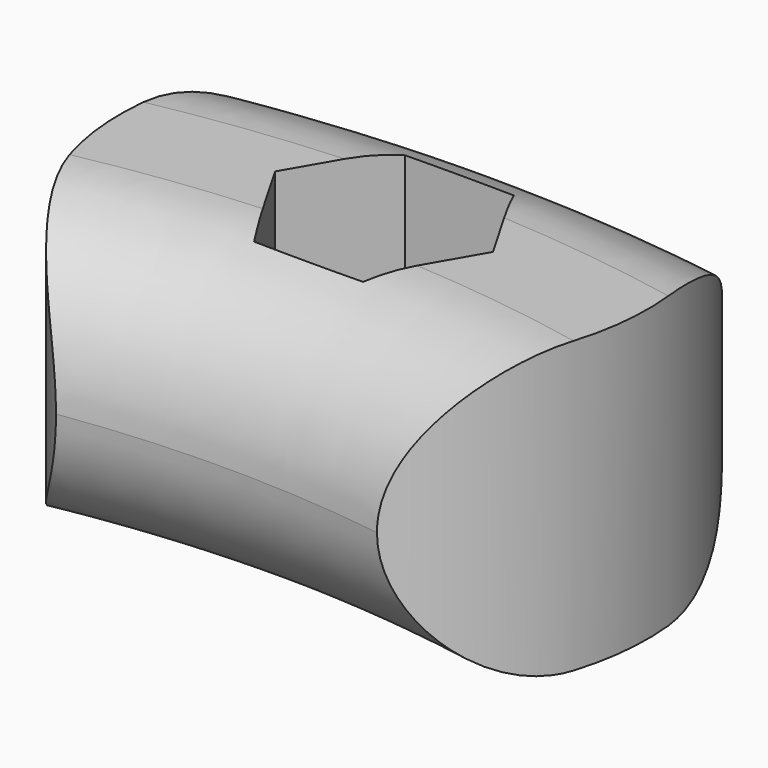
from build123d import *

# Parameters (mm, degrees)
F0_W     = 15
F0_H     = 11
F3_DEPTH = 8.5
F5_R     = 10
F6_DEPTH = 25


# Not quite as in the source:
# - a fillet or chamfer that OpenCascade refuses, or shapes differently, is made with other operations: its cross-section is extruded or revolved along the edge and cut away or added


with BuildPart() as f1:
    # F0 (on Front) → F1 (revolve)
    with BuildSketch(Plane.XZ):
        with Locations((50, 5.5)):
            Rectangle(F0_W, F0_H)
    revolve(axis=Axis((0, 0, 11.3872010261), (0, 0, 1)))

    # F2 (on face) → F3 (cut)
    with BuildSketch(Plane.XY.offset(11)):
        Polygon((-2.0640272124, 46.425), (2.0640272124, 46.425), (4.1280544247, 50), (2.0640272124, 53.575), (-2.0640272124, 53.575), (-4.1280544247, 50), align=None)
        Polygon((-15.8591658515, 43.680976315), (-15.3203466262, 47.7737146618), (-18.5953523929, 50.2867149724), (-22.409177385, 48.7069769362), (-22.9479966103, 44.6142385893), (-19.6729908436, 42.1012382787), align=None)
        Polygon((-31.3679446782, 34.286919955), (-32.4363637825, 38.2743143361), (-36.4237581637, 39.3427334405), (-39.3427334405, 36.4237581637), (-38.2743143361, 32.4363637825), (-34.286919955, 31.3679446782), align=None)
        Polygon((-42.1012382787, 19.6729908436), (-44.6142385893, 22.9479966103), (-48.7069769362, 22.409177385), (-50.2867149724, 18.5953523929), (-47.7737146618, 15.3203466262), (-43.680976315, 15.8591658515), align=None)
        Polygon((-46.425, 2.0640272124), (-50, 4.1280544247), (-53.575, 2.0640272124), (-53.575, -2.0640272124), (-50, -4.1280544247), (-46.425, -2.0640272124), align=None)
        Polygon((-43.680976315, -15.8591658515), (-47.7737146618, -15.3203466262), (-50.2867149724, -18.5953523929), (-48.7069769362, -22.409177385), (-44.6142385893, -22.9479966103), (-42.1012382787, -19.6729908436), align=None)
        Polygon((-34.286919955, -31.3679446782), (-38.2743143361, -32.4363637825), (-39.3427334405, -36.4237581637), (-36.4237581637, -39.3427334405), (-32.4363637825, -38.2743143361), (-31.3679446782, -34.286919955), align=None)
        Polygon((-19.6729908436, -42.1012382787), (-22.9479966103, -44.6142385893), (-22.409177385, -48.7069769362), (-18.5953523929, -50.2867149724), (-15.3203466262, -47.7737146618), (-15.8591658515, -43.680976315), align=None)
        Polygon((-2.0640272124, -46.425), (-4.1280544247, -50), (-2.0640272124, -53.575), (2.0640272124, -53.575), (4.1280544247, -50), (2.0640272124, -46.425), align=None)
        Polygon((15.8591658515, -43.680976315), (15.3203466262, -47.7737146618), (18.5953523929, -50.2867149724), (22.409177385, -48.7069769362), (22.9479966103, -44.6142385893), (19.6729908436, -42.1012382787), align=None)
        Polygon((31.3679446782, -34.286919955), (32.4363637825, -38.2743143361), (36.4237581637, -39.3427334405), (39.3427334405, -36.4237581637), (38.2743143361, -32.4363637825), (34.286919955, -31.3679446782), align=None)
        Polygon((42.1012382787, -19.6729908436), (44.6142385893, -22.9479966103), (48.7069769362, -22.409177385), (50.2867149724, -18.5953523929), (47.7737146618, -15.3203466262), (43.680976315, -15.8591658515), align=None)
        Polygon((46.425, -2.0640272124), (50, -4.1280544247), (53.575, -2.0640272124), (53.575, 2.0640272124), (50, 4.1280544247), (46.425, 2.0640272124), align=None)
        Polygon((43.680976315, 15.8591658515), (47.7737146618, 15.3203466262), (50.2867149724, 18.5953523929), (48.7069769362, 22.409177385), (44.6142385893, 22.9479966103), (42.1012382787, 19.6729908436), align=None)
        Polygon((34.286919955, 31.3679446782), (38.2743143361, 32.4363637825), (39.3427334405, 36.4237581637), (36.4237581637, 39.3427334405), (32.4363637825, 38.2743143361), (31.3679446782, 34.286919955), align=None)
        Polygon((19.6729908436, 42.1012382787), (22.9479966103, 44.6142385893), (22.409177385, 48.7069769362), (18.5953523929, 50.2867149724), (15.3203466262, 47.7737146618), (15.8591658515, 43.680976315), align=None)
    extrude(amount=-F3_DEPTH, mode=Mode.SUBTRACT)

    # F4: fillet of radius 5.5 on 4 edges, made by hand

    # F4_s1 → F4_t2 (revolve, cut)
    with BuildSketch(Plane.XZ):
        with BuildLine():
            ThreePointArc((48, 11), (44.1109127035, 9.3890872965), (42.5, 5.5))
            Line((42.5, 5.5), (42.5, 11))
            Line((42.5, 11), (48, 11))
        make_face()
    revolve(axis=Axis((0, 0, 11), (0, 0, 1)), mode=Mode.SUBTRACT)

    # F4_s3 → F4_t4 (revolve, cut)
    with BuildSketch(Plane.XZ):
        with BuildLine():
            ThreePointArc((52, 11), (55.8890872965, 9.3890872965), (57.5, 5.5))
            Line((57.5, 5.5), (57.5, 11))
            Line((57.5, 11), (52, 11))
        make_face()
    revolve(axis=Axis((0, 0, 11), (0, 0, 1)), mode=Mode.SUBTRACT)

    # F4_s5 → F4_t6 (revolve, cut)
    with BuildSketch(Plane.XZ):
        with BuildLine():
            ThreePointArc((57.5, 5.5), (55.8890872965, 1.6109127035), (52, 0))
            Line((52, 0), (57.5, 0))
            Line((57.5, 0), (57.5, 5.5))
        make_face()
    revolve(axis=Axis((0, 0, 0), (0, 0, 1)), mode=Mode.SUBTRACT)

    # F4_s7 → F4_t8 (revolve, cut)
    with BuildSketch(Plane.XZ):
        with BuildLine():
            ThreePointArc((42.5, 5.5), (44.1109127035, 1.6109127035), (48, 0))
            Line((48, 0), (42.5, 0))
            Line((42.5, 0), (42.5, 5.5))
        make_face()
    revolve(axis=Axis((0, 0, 0), (0, 0, 1)), mode=Mode.SUBTRACT)


with BuildPart() as f6:
    # F5 (on Top) → F6 (new body)
    with BuildSketch(Plane.XY):
        with Locations((0, 50)):
            Circle(F5_R)
    extrude(amount=F6_DEPTH)

    # F7: intersect F1
    add(f1.part, mode=Mode.INTERSECT)


solid = f6.part
